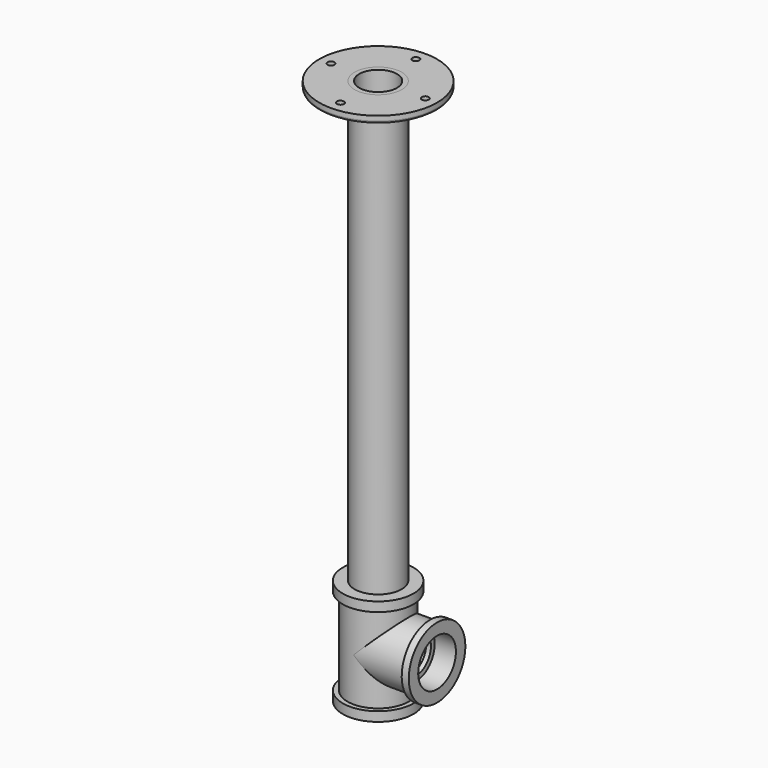
from build123d import *

# Parameters (mm, degrees)
F0_W           = 2.54
F0_H           = 254
F9_D           = 3.81
F9_CSINK_D     = 6.35
F9_CSINK_ANGLE = 90


with BuildPart() as f1:
    # F0 (on Front) → F1 (revolve)
    with BuildSketch(Plane.XZ):
        with Locations((11.43, -127)):
            Rectangle(F0_W, F0_H)
    revolve(axis=Axis((0, 0, -67.6468755098), (0, 0, -1)))


with BuildPart() as f3:
    # F2 (on Front) → F3 (revolve)
    with BuildSketch(Plane.XZ):
        with BuildLine():
            Line((12.7, 0), (12.7, -9.525))
            Line((12.7, -9.525), (16.256, -9.525))
            ThreePointArc((16.256, -9.525), (16.4356051224, -9.4506051224), (16.51, -9.271))
            Line((16.51, -9.271), (16.51, -6.35))
            ThreePointArc((16.51, -6.35), (17.2539487758, -4.5539487758), (19.05, -3.81))
            Line((19.05, -3.81), (30.48, -3.81))
            ThreePointArc((30.48, -3.81), (31.3780256121, -3.4380256121), (31.75, -2.54))
            Line((31.75, -2.54), (31.75, 0))
            Line((31.75, 0), (12.7, 0))
        make_face()
    revolve(axis=Axis((0, 0, -110.5323322117), (0, 0, -1)))

    # F9 (through all)
    with Locations(Plane(origin=(0, 0, -3.81), x_dir=(1, 0, 0), z_dir=(0, 0, -1))):
        with Locations((25.4, 0), (0, 25.4), (-25.4, 0), (0, -25.4)):
            CounterSinkHole(F9_D / 2, F9_CSINK_D / 2, counter_sink_angle=F9_CSINK_ANGLE)


with BuildPart() as f5:
    # F4 (on Front) → F5 (revolve)
    with BuildSketch(Plane.XZ):
        Polygon((19.05, -236.9874591094), (12.7, -236.9874591094), (12.7, -248.4174591094), (11.4581380039, -248.4174591094), (11.43, -250.9573032489), (12.7, -250.9573032489), (12.7, -280.1674591094), (11.43, -280.1674591094), (11.43, -282.7074591094), (12.7, -282.7074591094), (12.7, -294.1374591094), (19.05, -294.1374591094), (19.05, -289.0574591094), (16.51, -289.0574591094), (16.51, -242.0674591094), (19.05, -242.0674591094), align=None)
    revolve(axis=Axis((0, 0, -105.1599124395), (0, 0, -1)))

    # F6 (on Front) → F7 (revolve)
    with BuildSketch(Plane.XZ):
        Polygon((0, -249.0524591094), (0, -252.8624591094), (17.78, -252.8624591094), (17.78, -255.4024591094), (20.32, -255.4024591094), (20.32, -252.8624591094), (31.75, -252.8624591094), (31.75, -246.5124591094), (27.94, -246.5124591094), (27.94, -249.0524591094), align=None)
    revolve(axis=Axis((24.5970338583, 0, -265.5624591094), (1, 0, 0)))


solid = Compound([f1.part, f3.part, f5.part])
